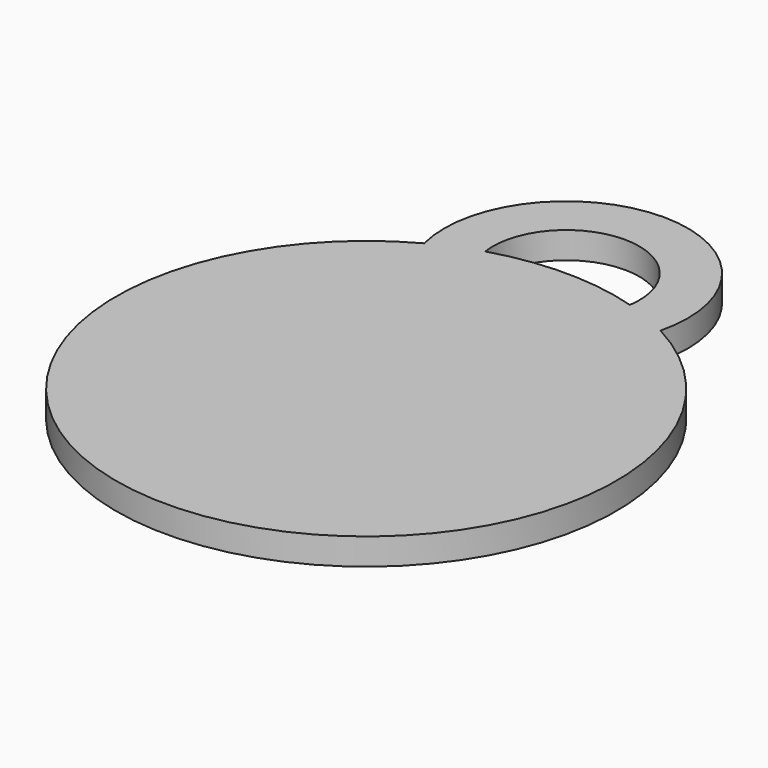
from build123d import *

# Parameters (mm, degrees)
F1_DEPTH = 6.35


# Not quite as in the source:
# - the program builds the solid bodies; features that only make, move or delete a surface that nothing else refers to are left out


with BuildPart() as f1:
    # F0 (on Top) → F1 (new body)
    with BuildSketch(Plane.XY):
        with BuildLine():
            ThreePointArc((-28.1745800825, 52.5502901658), (0, -59.6266715433), (28.1745800825, 52.5502901658))
            ThreePointArc((28.1745800825, 52.5502901658), (0, 88.6763210459), (-28.1745800825, 52.5502901658))
        make_face()
        with BuildLine():
            ThreePointArc((-17.2520936805, 57.0763105235), (0, 77.0662551877), (17.2520936805, 57.0763105235))
            ThreePointArc((17.2520936805, 57.0763105235), (0, 59.6266715433), (-17.2520936805, 57.0763105235))
        make_face(mode=Mode.SUBTRACT)
    extrude(amount=F1_DEPTH)


solid = f1.part
